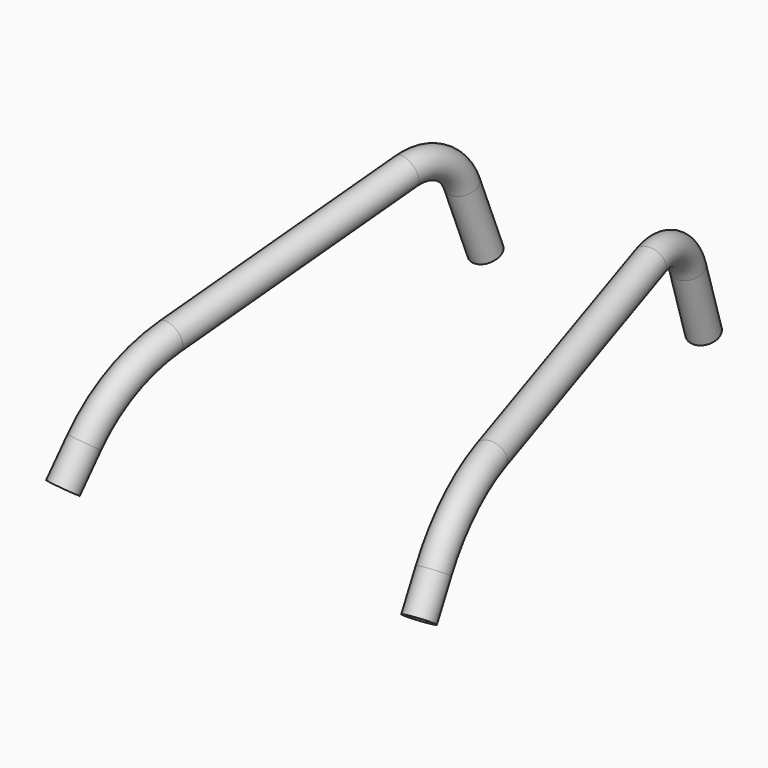
from build123d import *

# Parameters (mm, degrees)
F6_R   = 28.575
F6_R_2 = 25.8


# Not quite as in the source:
# - a pattern or mirror of a feature is missing from the dataset's text; its kind, count and spacing are read off the source's solid


with BuildPart() as f7:
    # F7: sweep along a path in F4
    with BuildLine(Plane(origin=(219.6377502383, 34.3183984747, 0), x_dir=(0.1543768803, -0.9880120338, 0), z_dir=(-0.9880120338, -0.1543768803, 0))) as f7_path:
        Line((844.4415350966, -0.0045336783), (799.7197425418, 63.8648052169))
        ThreePointArc((799.7197425418, 63.8648052169), (721.7320002963, 140.5031460781), (621.4594455582, 184.1028937472))
        Line((621.4594455582, 184.1028937472), (130.575108047, 297.4324728002))
        ThreePointArc((130.575108047, 297.4324728002), (60.3641265867, 287.8771775879), (14.1107405341, 234.1974806543))
        Line((14.1107405341, 234.1974806543), (-34.7347980616, 99.9954663217))
    # F6 (on line) → F7 (sweep)
    with BuildSketch(Plane(origin=(42.8881960501, -274.4844547207, -396.7607817515), x_dir=(0.9960720051, 0.0503774711, 0.072819442), z_dir=(-0.0885469408, 0.5667004214, 0.8191520443))):
        with Locations((308.3228947197, -657.9033070538)):
            Circle(F6_R)
        with Locations((308.3228947197, -657.9033070538)):
            Circle(F6_R_2, mode=Mode.SUBTRACT)
    sweep(path=f7_path.line)


with BuildPart() as f7_copies_1:
    # F7_copies: instance of F7
    add(f7.part.mirror(Plane(origin=(0, 0, 0), x_dir=(0, 0, -1), z_dir=(-1, 0, 0))))


solid = Compound([f7.part, f7_copies_1.part])
